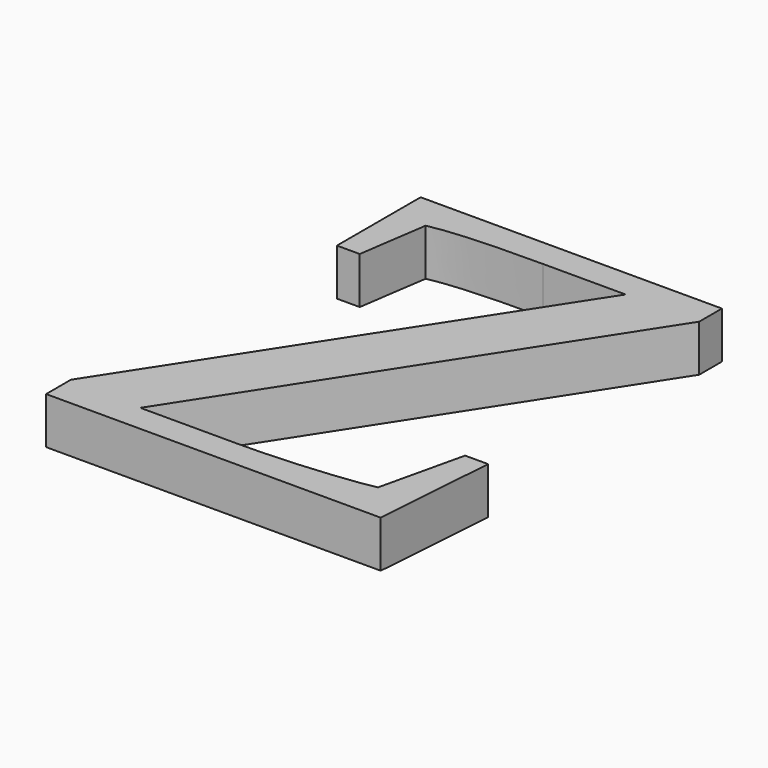
from build123d import *

# Parameters (mm, degrees)
F0_TEXT_SIZE = 144.6309809883
F1_DEPTH     = 10


# Not quite as in the source:
# - Text() gives the source's letters only with a copy of the font that has no kerning and outlines rounded to 1/6400 em; it was checked with that copy


with BuildPart() as f1:
    # F0 (on Top) → F1 (new body)
    with BuildSketch(Plane.XY):
        with Locations((-70.801615715, -45.5835536122)):
            Text('Z', F0_TEXT_SIZE, font='Tinos', text_align=(TextAlign.LEFT, TextAlign.BOTTOM))
    extrude(amount=F1_DEPTH)


solid = f1.part
